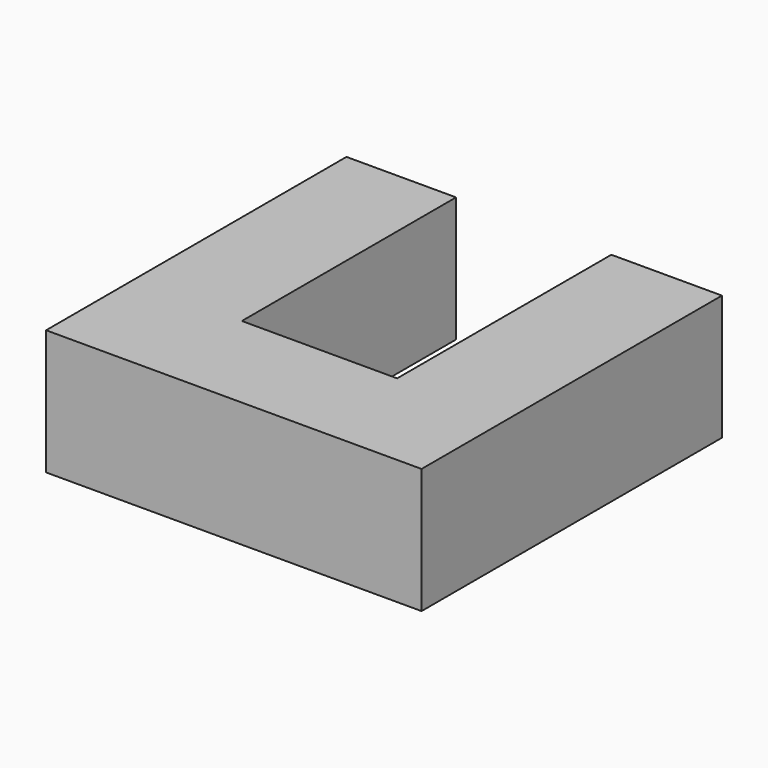
from build123d import *

# Parameters (mm, degrees)
F1_DEPTH = 25.4
F3_DEPTH = 25.4


# Not quite as in the source:
# - a feature names something its author has since deleted; it is built from what else it names


with BuildPart() as f1:
    # F0 (on Top) → F1 (new body)
    with BuildSketch(Plane.XY):
        Polygon((-27.94, 43.9866697311), (-53.755334568, 43.9866697311), (-53.755334568, -32.2133302689), (22.444665432, -32.2133302689), (22.444665432, 43.9866697311), (0, 43.9866697311), (0, 5.8866697311), (-27.94, 5.8866697311), align=None)
    extrude(amount=F1_DEPTH)

    # F2 (on face) → F3 (cut)
    with BuildSketch(Plane.XY.offset(25.4)):
        Polygon((-27.94, 43.9866697311), (-31.5155684948, 43.9866697311), (-31.5155684948, 0), (-31.5155684948, -10.3501314297), (0, -10.3501314297), (0, 5.8866697311), (-27.94, 5.8866697311), align=None)
    extrude(amount=-F3_DEPTH, mode=Mode.SUBTRACT)


solid = f1.part
